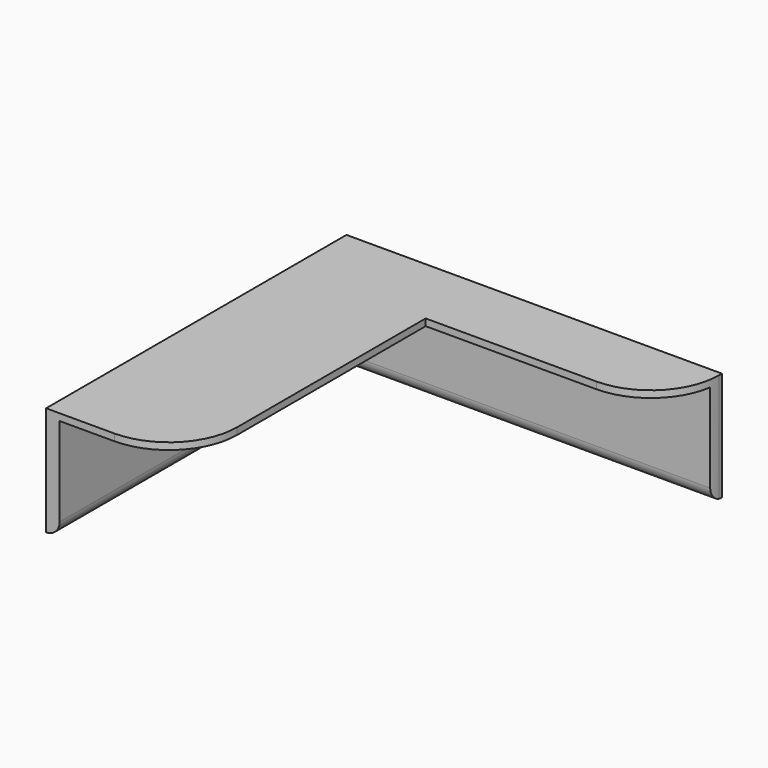
from build123d import *

# Parameters (mm, degrees)
F1_DEPTH     = 1
F3_DEPTH     = 15
F4_R         = 1.99999
F5_R         = 10
F6_TEXT_SIZE = 5.3872960824
F7_DEPTH     = 0.3


# Not quite as in the source:
# - a fillet or chamfer is up to 0.001 mm smaller than in the source, because OpenCascade refuses the exact size
# - Text() gives the source's letters only with a copy of the font that has no kerning and outlines rounded to 1/6400 em; it was checked with that copy


with BuildPart() as f1:
    # F0 (on Top) → F1 (new body)
    with BuildSketch(Plane.XY):
        Polygon((-20, -44.5), (0, -44.5), (0, 0), (35, 0), (35, 10.5), (-20, 10.5), (-20, 0), align=None)
    extrude(amount=F1_DEPTH)

    # F2 (on face) → F3 (join)
    with BuildSketch(Plane(origin=(0, 0, 0), x_dir=(1, 0, 0), z_dir=(0, 0, -1))):
        Polygon((-20, 44.5), (-20, -10.5), (-18, -10.5), (35, -10.5), (35, -8.5), (-18, -8.5), (-18, 44.5), align=None)
    extrude(amount=F3_DEPTH)

    # F4 (radius 2 in the source; OpenCascade refuses exactly that, so slightly less here)
    f4_edges = [f1.edges().sort_by_distance(p)[0] for p in [
        (-18, -18, -15),
        (8.5, 8.5, -15),
    ]]
    fillet(f4_edges, radius=F4_R)

    # F5
    f5_edges = [f1.edges().sort_by_distance(p)[0] for p in [
        (0, -44.5, 0.5),
        (35, 0, 0.5),
    ]]
    fillet(f5_edges, radius=F5_R)

    # F6 (on face) → F7 (join)
    with BuildSketch(Plane(origin=(-20, 0, 0), x_dir=(0, -1, 0), z_dir=(-1, 0, 0))):
        with Locations((-8, -8.8788531793)):
            Text('Etikettmall  - Wera', F6_TEXT_SIZE, font='Open Sans', font_style=FontStyle.BOLD, text_align=(TextAlign.LEFT, TextAlign.BOTTOM))
    extrude(amount=F7_DEPTH)


solid = f1.part
